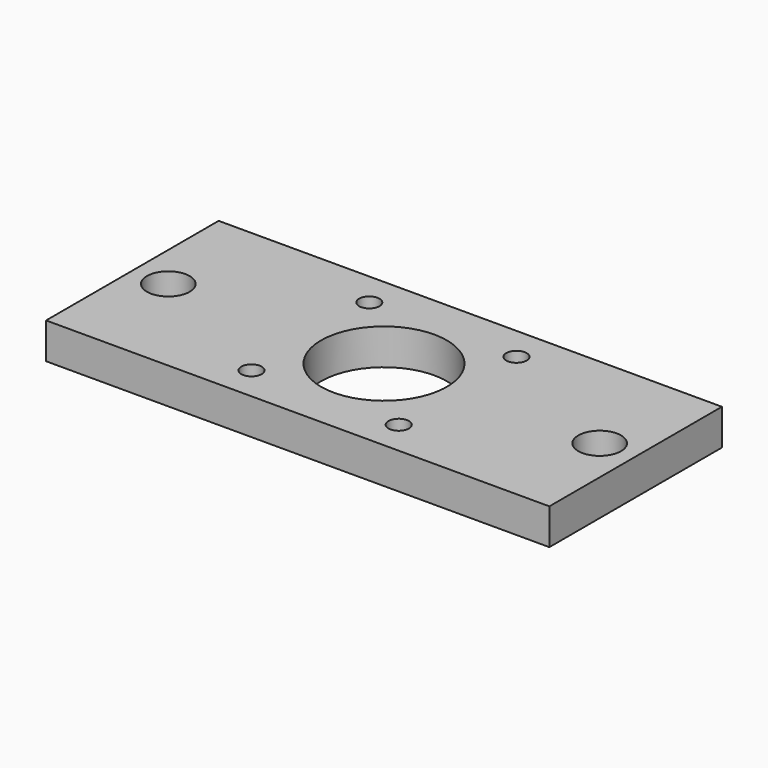
from build123d import *

# Parameters (mm, degrees)
F1_DEPTH = 6.35
F2_D     = 3.6
F3_D     = 7.5438
F4_D     = 22.225


# Not quite as in the source:
# - a length typed as a fraction of an inch, garbled in the dataset ("3 / 203.2 mm" for 3/8 in), is restored


with BuildPart() as f1:
    # F0 (on Top) → F1 (new body)
    with BuildSketch(Plane.XY):
        Polygon((44.45, 13), (44.45, 19.05), (-44.45, 19.05), (-44.45, -19.05), (44.45, -19.05), align=None)
    extrude(amount=F1_DEPTH)

    # F2 (through all)
    with Locations(Plane(origin=(0, 0, 0), x_dir=(1, 0, 0), z_dir=(0, 0, -1))):
        with Locations((-13, -13), (13, -13), (13, 13), (-13, 13)):
            Hole(F2_D / 2)

    # F3 (through all)
    with Locations(Plane(origin=(0, 0, 0), x_dir=(1, 0, 0), z_dir=(0, 0, -1))):
        with Locations((-38.1, 0), (38.1, 0)):
            Hole(F3_D / 2)

    # F4 (through all)
    with Locations(Plane(origin=(0, 0, 0), x_dir=(1, 0, 0), z_dir=(0, 0, -1))):
        with Locations((0, 0)):
            Hole(F4_D / 2)


solid = f1.part
